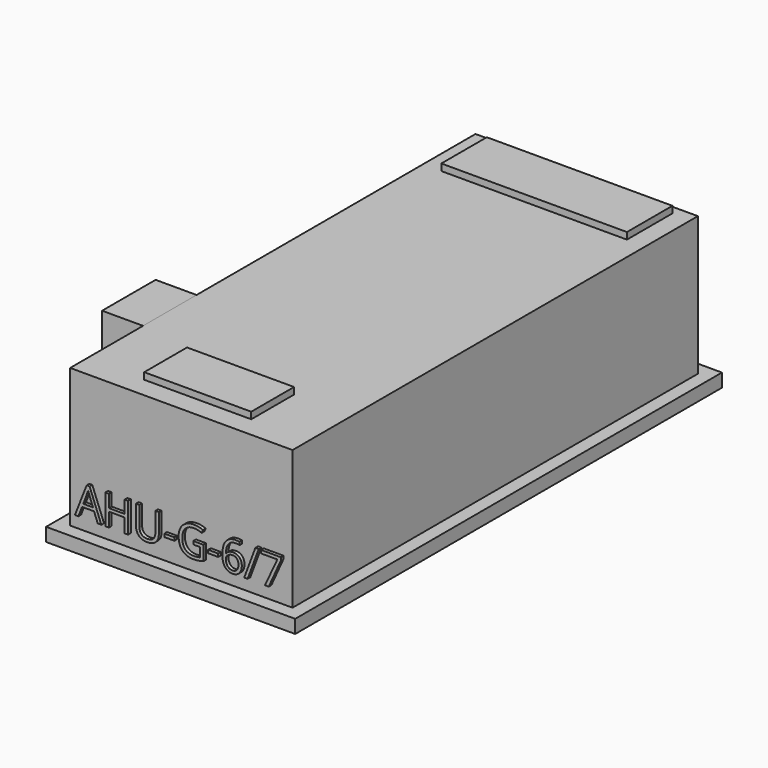
from build123d import *

# Parameters (mm, degrees)
F0_W         = 1689.1
F0_H         = 1054.1
F1_DEPTH     = 3848.1
F2_W         = 1892.3
F2_H         = 101.6
F3_DEPTH     = 3949.7
F4_DEPTH     = 101.6
F5_W         = 812.8
F5_H         = 406.4
F6_DEPTH     = 50.8
F7_W         = 508
F7_H         = 762
F8_DEPTH     = 311.15
F9_TEXT_SIZE = 317.5
F10_DEPTH    = 25.4
F11_W        = 1409.7
F11_H        = 431.8
F12_DEPTH    = 50.8
F13_W        = 1409.7
F13_H        = 431.8
F14_DEPTH    = 50.8


# Not quite as in the source:
# - Text() gives the source's letters only with a copy of the font that has no kerning and outlines rounded to 1/6400 em; it was checked with that copy


with BuildPart() as f1:
    # F0 (on Front) → F1 (new body)
    with BuildSketch(Plane.XZ):
        with Locations((204.6098696411, -25.3882179465)):
            Rectangle(F0_W, F0_H)
    extrude(amount=F1_DEPTH)

    # F5 (on face) → F6 (join)
    with BuildSketch(Plane.XY.offset(501.6617820535)):
        with Locations((204.6098696411, -3489.325)):
            Rectangle(F5_W, F5_H)
    extrude(amount=F6_DEPTH)

    # F9 (on face) → F10 (join)
    with BuildSketch(Plane.XZ.offset(3848.1)):
        with Locations((-583.7821622895, -453.3843984417)):
            Text('AHU-G-6/7', F9_TEXT_SIZE, font='Open Sans', text_align=(TextAlign.LEFT, TextAlign.BOTTOM))
    extrude(amount=F10_DEPTH)

    # F11 (on face) → F12 (join)
    with BuildSketch(Plane.XY.offset(501.6617820535)):
        with Locations((204.6098696411, -282.575)):
            Rectangle(F11_W, F11_H)
    extrude(amount=F12_DEPTH)

    # F13 (on face) → F14 (join)
    with BuildSketch(Plane(origin=(0, 0, 0), x_dir=(-1, 0, 0), z_dir=(0, 1, 0))):
        with Locations((-204.6098696411, 9.5367820535)):
            Rectangle(F13_W, F13_H)
    extrude(amount=F14_DEPTH)


with BuildPart() as f3:
    # F2 (on face) → F3 (new body)
    with BuildSketch(Plane.XZ.offset(3848.1)):
        with Locations((204.6098696411, -603.2382179465)):
            Rectangle(F2_W, F2_H)
    extrude(amount=-F3_DEPTH)

    # F4 (add): a face of the model
    f4_faces = [f3.faces().sort_by_distance(p)[0] for p in [
        (204.6098696411, -3848.1, -603.2382179465),
    ]]
    extrude(f4_faces, amount=F4_DEPTH)


with BuildPart() as f8:
    # F7 (on face) → F8 (new body)
    with BuildSketch(Plane(origin=(-639.9401303589, 0, 0), x_dir=(0, -1, 0), z_dir=(-1, 0, 0))):
        with Locations((2901.95, 120.6617820535)):
            Rectangle(F7_W, F7_H)
    extrude(amount=F8_DEPTH)


solid = Compound([f1.part, f3.part, f8.part])
